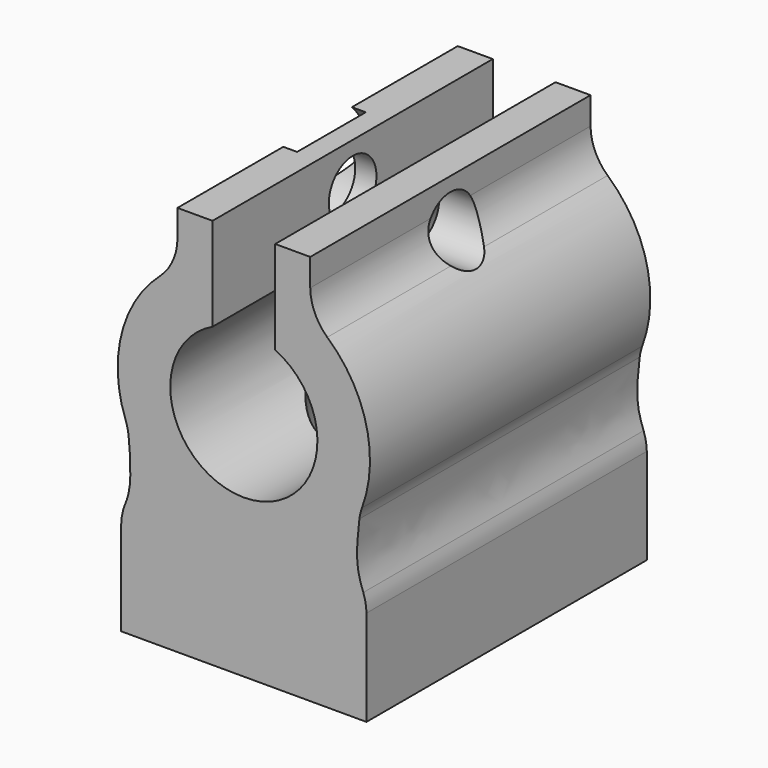
from build123d import *

# Parameters (mm, degrees)
F1_DEPTH     = 20
F2_R         = 3.5
F2_R_2       = 1.7
F3_DEPTH     = 4
F4_DEPTH     = 25
F5_T1_DEPTH  = 20
F5_T6_DEPTH  = 12.1022846539
F5_S7_R      = 1.7
F5_T8_DEPTH  = 8
F5_T12_DEPTH = 12.1022846539
F5_S13_R     = 1.7
F5_T14_DEPTH = 8
F5_T18_DEPTH = 10.2630041323
F5_S19_R     = 3.5
F5_T20_DEPTH = 7
F5_T24_DEPTH = 10.2630041323
F5_S25_R     = 3.5
F5_T26_DEPTH = 7
F5_T27_DEPTH = 23.3663915102
F5_T29_DEPTH = 22.9020360067
F6_R         = 3.5
F6_R_2       = 1.7
F7_DEPTH     = 12
F8_DEPTH     = 12
F9_DEPTH     = 6


# Not quite as in the source:
# - a fillet or chamfer that OpenCascade refuses, or shapes differently, is made with other operations: its cross-section is extruded or revolved along the edge and cut away or added


with BuildPart() as f1:
    # F0 (on Front) → F1 (new body)
    with BuildSketch(Plane.XZ):
        with BuildLine():
            ThreePointArc((1.7894736842, 3.7997084011), (0, -4.2), (-1.7894736842, 3.7997084011))
            Line((-1.7894736842, 3.7997084011), (-1.7894736842, 9.1220820965))
            Line((-1.7894736842, 9.1220820965), (-3.7894736842, 9.1220820965))
            Line((-3.7894736842, 9.1220820965), (-3.7894736842, 6.1220820965))
            ThreePointArc((-3.7894736842, 6.1220820965), (-6.8557776995, 2.199616361), (-6.6439040907, -2.7746240166))
            add(Edge.make_bspline(
                [(-6.6356726702, -2.7942527112), (-6.6390399212, -2.7803089062), (-6.6413283577, -2.7774058988), (-6.6439040907, -2.7746240166)],
                knots=[0.9532514843, 0.9532514843, 0.9532514843, 0.9532514843, 1, 1, 1, 1], degree=3))
            add(Edge.make_bspline(
                [(-7, -7.2), (-6.7795680226, -6.7700727801), (-6.2785456929, -5.7974600377), (-6.5973790049, -2.9528269921), (-6.6356726702, -2.7942527112)],
                knots=[0, 0, 0, 0, 0.4216094964, 0.9532514843, 0.9532514843, 0.9532514843, 0.9532514843], degree=3))
            Line((-7, -7.2), (-7, -13.2))
            Line((-7, -13.2), (7, -13.2))
            Line((7, -13.2), (7, -7.2))
            add(Edge.make_bspline(
                [(7, -7.2), (6.7871491537, -6.6864508711), (6.3058923114, -5.5253136877), (6.5175995563, -3.7720698099), (6.6356726702, -2.7942527112)],
                knots=[0, 0, 0, 0, 0.4422811845, 1, 1, 1, 1], degree=3))
            ThreePointArc((6.6356726702, -2.7942527112), (6.8590214848, 2.1894803656), (3.7894736842, 6.1220820965))
            Line((3.7894736842, 6.1220820965), (3.7894736842, 9.1220820965))
            Line((3.7894736842, 9.1220820965), (1.7894736842, 9.1220820965))
            Line((1.7894736842, 9.1220820965), (1.7894736842, 3.7997084011))
        make_face()
        with BuildLine():
            add(Edge.make_bspline(
                [(-6.6356726702, -2.7942527112), (-6.6390399212, -2.7803089062), (-6.6413283577, -2.7774058988), (-6.6439040907, -2.7746240166)],
                knots=[0.9532514843, 0.9532514843, 0.9532514843, 0.9532514843, 1, 1, 1, 1], degree=3))
            ThreePointArc((-6.6439040907, -2.7746240166), (-6.6397956338, -2.7844414056), (-6.6356726702, -2.7942527112))
        make_face()
    extrude(amount=F1_DEPTH)

    # F2 (on face) → F3 (cut)
    with BuildSketch(Plane(origin=(-7, 0, 0), x_dir=(0, -1, 0), z_dir=(-1, 0, 0))):
        with Locations((10, 6.622)):
            Circle(F2_R)
        with Locations((10, 6.622)):
            Circle(F2_R_2, mode=Mode.SUBTRACT)
    extrude(amount=-F3_DEPTH, mode=Mode.SUBTRACT)

    # F2 (on face) → F4 (cut)
    with BuildSketch(Plane(origin=(-7, 0, 0), x_dir=(0, -1, 0), z_dir=(-1, 0, 0))):
        with Locations((10, 6.622)):
            Circle(F2_R_2)
    extrude(amount=-F4_DEPTH, mode=Mode.SUBTRACT)

    # F5: fillet of radius 3 on 8 edges, made by hand

    # F5_s2 → F5_t1 (join)
    with BuildSketch(Plane.XZ):
        with BuildLine():
            ThreePointArc((-6.5767127025, -3.2402461743), (-6.6395606645, -2.8691274316), (-6.7483493849, -2.5087886996))
            Line((-6.7483493849, -2.5087886996), (-6.466927581, -2.4041663985))
            ThreePointArc((-6.466927581, -2.4041663985), (-6.4145893512, -2.5416001874), (-6.3589651198, -2.6777323732))
            Line((-6.3589651198, -2.6777323732), (-6.343821894, -2.723774473))
            ThreePointArc((-6.343821894, -2.723774473), (-6.304537605, -2.9799785061), (-6.2781272304, -3.2087696206))
            Line((-6.2781272304, -3.2087696206), (-6.5767127025, -3.2402461743))
        make_face()
        with BuildLine():
            ThreePointArc((6.5887317904, -3.1834061265), (6.6509501418, -2.8334452349), (6.754091056, -2.4932898281))
            Line((6.754091056, -2.4932898281), (6.4724298111, -2.3893138658))
            ThreePointArc((6.4724298111, -2.3893138658), (6.4175024363, -2.534235691), (6.3589651198, -2.6777323732))
            Line((6.3589651198, -2.6777323732), (6.3375979172, -2.7582596669))
            ThreePointArc((6.3375979172, -2.7582596669), (6.3141276632, -2.9530960278), (6.290534619, -3.1484417941))
            Line((6.290534619, -3.1484417941), (6.5887317904, -3.1834061265))
        make_face()
    extrude(amount=F5_T1_DEPTH)


with BuildPart() as f5_tool4:
    # F5_s5 → F5_t6 (new body)
    with BuildSketch(Plane.XZ.offset(7.8977153461)):
        with BuildLine():
            ThreePointArc((4.792775332, 5.3724803189), (4.0514647707, 6.385428811), (3.7890736842, 7.6129290813))
            Line((3.7890736842, 7.6129290813), (3.4888336842, 7.6129290813))
            ThreePointArc((3.4888336842, 7.6129290813), (3.4892336842, 6.8675055889), (3.4892336842, 6.1220820965))
            Line((3.4892336842, 6.1220820965), (3.6314526316, 5.8667912731))
            ThreePointArc((3.6314526316, 5.8667912731), (4.1279416848, 5.5287236777), (4.5929054968, 5.1484354427))
            Line((4.5929054968, 5.1484354427), (4.792775332, 5.3724803189))
        make_face()
    extrude(amount=F5_T6_DEPTH)

    # F5_s7 → F5_t8 (cut, symmetric)
    with BuildSketch(Plane.YZ.offset(4.1)):
        with Locations((-10, 6.622)):
            Circle(F5_S7_R)
    extrude(amount=F5_T8_DEPTH, both=True, mode=Mode.SUBTRACT)


with BuildPart() as f1_1:
    add(f1.part)

    # F5_t3: union F5_tool4
    add(f5_tool4.part)


with BuildPart() as f5_tool10:
    # F5_s11 → F5_t12 (new body)
    with BuildSketch(Plane.XZ):
        with BuildLine():
            ThreePointArc((4.792775332, 5.3724803189), (4.0514647707, 6.385428811), (3.7890736842, 7.6129290813))
            Line((3.7890736842, 7.6129290813), (3.4888336842, 7.6129290813))
            ThreePointArc((3.4888336842, 7.6129290813), (3.4892336842, 6.8675055889), (3.4892336842, 6.1220820965))
            Line((3.4892336842, 6.1220820965), (3.6314526316, 5.8667912731))
            ThreePointArc((3.6314526316, 5.8667912731), (4.1279416848, 5.5287236777), (4.5929054968, 5.1484354427))
            Line((4.5929054968, 5.1484354427), (4.792775332, 5.3724803189))
        make_face()
    extrude(amount=F5_T12_DEPTH)

    # F5_s13 → F5_t14 (cut, symmetric)
    with BuildSketch(Plane.YZ.offset(4.1)):
        with Locations((-10, 6.622)):
            Circle(F5_S13_R)
    extrude(amount=F5_T14_DEPTH, both=True, mode=Mode.SUBTRACT)


with BuildPart() as f1_2:
    add(f1_1.part)

    # F5_t9: union F5_tool10
    add(f5_tool10.part)


with BuildPart() as f5_tool16:
    # F5_s17 → F5_t18 (new body)
    with BuildSketch(Plane.XZ):
        with BuildLine():
            ThreePointArc((-3.7890736842, 7.6129290813), (-4.0514647707, 6.385428811), (-4.792775332, 5.3724803189))
            Line((-4.792775332, 5.3724803189), (-4.5929054968, 5.1484354427))
            ThreePointArc((-4.5929054968, 5.1484354427), (-4.1279416848, 5.5287236777), (-3.6314526316, 5.8667912731))
            Line((-3.6314526316, 5.8667912731), (-3.4892336842, 6.1220820965))
            ThreePointArc((-3.4892336842, 6.1220820965), (-3.4892336842, 6.8675055889), (-3.4888336842, 7.6129290813))
            Line((-3.4888336842, 7.6129290813), (-3.7890736842, 7.6129290813))
        make_face()
    extrude(amount=F5_T18_DEPTH)

    # F5_s19 → F5_t20 (cut, symmetric)
    with BuildSketch(Plane.YZ.offset(-4.1)):
        with Locations((-10, 6.622)):
            Circle(F5_S19_R)
    extrude(amount=F5_T20_DEPTH, both=True, mode=Mode.SUBTRACT)


with BuildPart() as f1_3:
    add(f1_2.part)

    # F5_t15: union F5_tool16
    add(f5_tool16.part)


with BuildPart() as f5_tool22:
    # F5_s23 → F5_t24 (new body)
    with BuildSketch(Plane.XZ.offset(9.7369958677)):
        with BuildLine():
            ThreePointArc((-4.792775332, 5.3724803189), (-4.0514647707, 6.385428811), (-3.7890736842, 7.6129290813))
            Line((-3.7890736842, 7.6129290813), (-3.4888336842, 7.6129290813))
            ThreePointArc((-3.4888336842, 7.6129290813), (-3.4892336842, 6.8675055889), (-3.4892336842, 6.1220820965))
            Line((-3.4892336842, 6.1220820965), (-3.6314526316, 5.8667912731))
            ThreePointArc((-3.6314526316, 5.8667912731), (-4.1279416848, 5.5287236777), (-4.5929054968, 5.1484354427))
            Line((-4.5929054968, 5.1484354427), (-4.792775332, 5.3724803189))
        make_face()
    extrude(amount=F5_T24_DEPTH)

    # F5_s25 → F5_t26 (cut, symmetric)
    with BuildSketch(Plane.YZ.offset(-4.1)):
        with Locations((-10, 6.622)):
            Circle(F5_S25_R)
    extrude(amount=F5_T26_DEPTH, both=True, mode=Mode.SUBTRACT)


with BuildPart() as f1_4:
    add(f1_3.part)

    # F5_t21: union F5_tool22
    add(f5_tool22.part)

    # F5_s28 → F5_t27 (cut)
    with BuildSketch(Plane.XZ.offset(-1.6831957551)):
        with BuildLine():
            ThreePointArc((-7.0004, -7.8732781832), (-6.9416848839, -7.2824101234), (-6.7678360085, -6.7146521667))
            Line((-6.7678360085, -6.7146521667), (-7.0448196093, -6.5987895651))
            ThreePointArc((-7.0448196093, -6.5987895651), (-7.148871707, -6.8283644641), (-7.2671697753, -7.0630169034))
            Line((-7.2671697753, -7.0630169034), (-7.30024, -7.2))
            ThreePointArc((-7.30024, -7.2), (-7.30024, -7.5366390916), (-7.30064, -7.8732781832))
            Line((-7.30064, -7.8732781832), (-7.0004, -7.8732781832))
        make_face()
    extrude(amount=F5_T27_DEPTH, mode=Mode.SUBTRACT)

    # F5_s30 → F5_t29 (cut)
    with BuildSketch(Plane.XZ.offset(-1.4510180034)):
        with BuildLine():
            ThreePointArc((7.0004, -7.7804070635), (6.9510099307, -7.2380620544), (6.8044646756, -6.7135604089))
            Line((6.8044646756, -6.7135604089), (7.0851111432, -6.6068757434))
            ThreePointArc((7.0851111432, -6.6068757434), (7.178454263, -6.8447161783), (7.277360411, -7.0850423555))
            Line((7.277360411, -7.0850423555), (7.30024, -7.2))
            ThreePointArc((7.30024, -7.2), (7.30024, -7.4902035318), (7.30064, -7.7804070635))
            Line((7.30064, -7.7804070635), (7.0004, -7.7804070635))
        make_face()
    extrude(amount=F5_T29_DEPTH, mode=Mode.SUBTRACT)

    # F6 (on face) → F7 (cut)
    with BuildSketch(Plane(origin=(0, 0, -13.2), x_dir=(1, 0, 0), z_dir=(0, 0, -1))):
        with Locations((0, 10)):
            Circle(F6_R)
        with Locations((0, 10)):
            Circle(F6_R_2, mode=Mode.SUBTRACT)
    extrude(amount=-F7_DEPTH, mode=Mode.SUBTRACT)

    # F8 (cut): a face of the model
    f8_faces = [f1_4.faces().sort_by_distance(p)[0] for p in [
        (0, -10, -13.2),
    ]]
    extrude(f8_faces, amount=-F8_DEPTH, mode=Mode.SUBTRACT)

    # F6 (on face) → F9 (join)
    with BuildSketch(Plane(origin=(0, 0, -13.2), x_dir=(1, 0, 0), z_dir=(0, 0, -1))):
        with Locations((0, 10)):
            Circle(F6_R)
        with Locations((0, 10)):
            Circle(F6_R_2, mode=Mode.SUBTRACT)
    extrude(amount=-F9_DEPTH)


solid = f1_4.part
